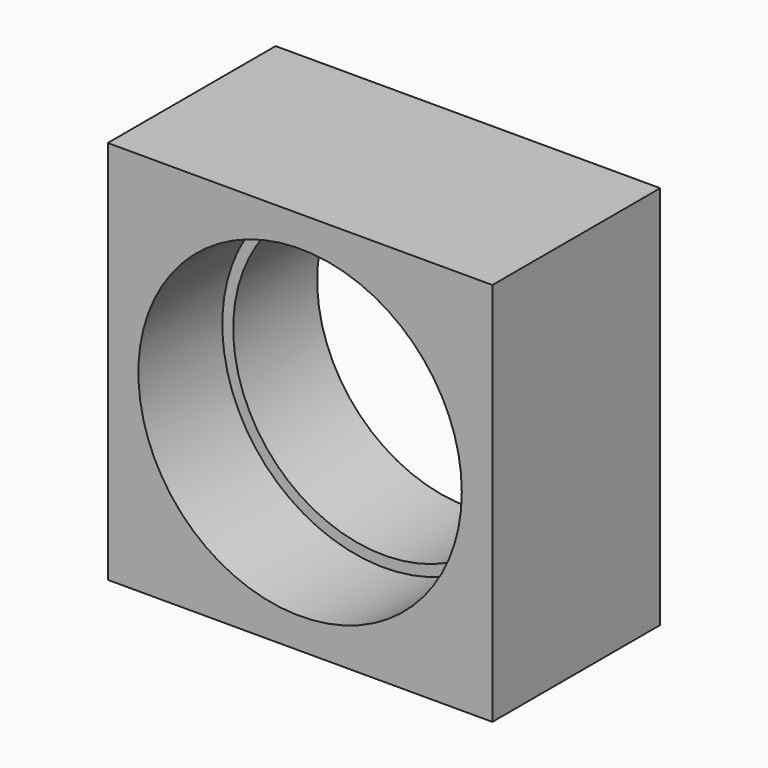
from build123d import *

# Parameters (mm, degrees)
F0_W     = 44
F0_H     = 44
F0_R     = 18.5
F1_DEPTH = 12
F2_W     = 44
F2_H     = 44
F2_R     = 17.25
F3_DEPTH = 12


# Not quite as in the source:
# - a feature names something its author has since deleted; it is built from what else it names


with BuildPart() as f1:
    # F0 (on Front) → F1 (new body)
    with BuildSketch(Plane.XZ):
        Rectangle(F0_W, F0_H)
        Circle(F0_R, mode=Mode.SUBTRACT)
    extrude(amount=F1_DEPTH)

    # F2 (on Front) → F3 (join)
    with BuildSketch(Plane.XZ):
        Rectangle(F2_W, F2_H)
        Circle(F2_R, mode=Mode.SUBTRACT)
    extrude(amount=-F3_DEPTH)


solid = f1.part
